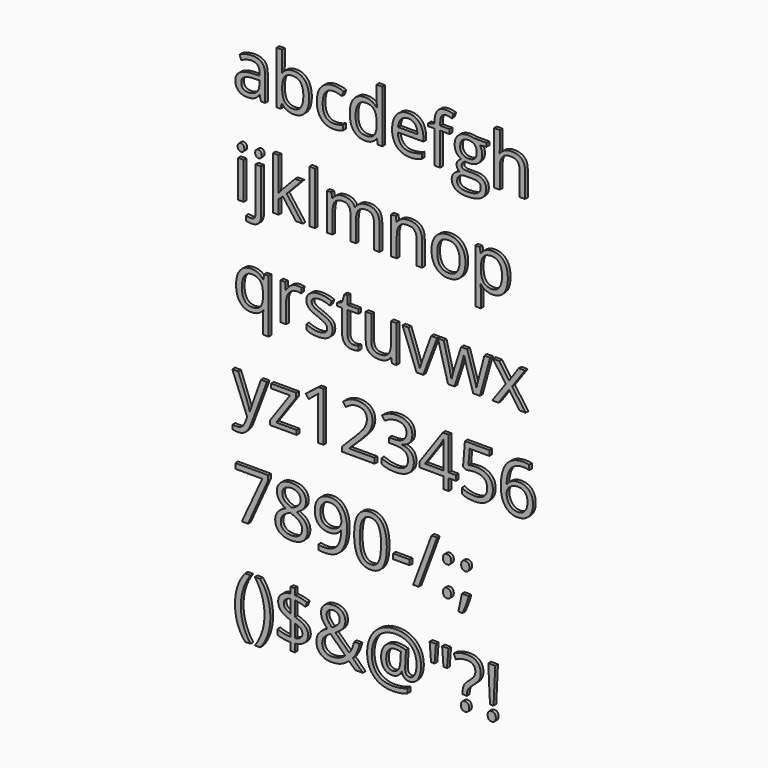
from build123d import *

# Parameters (mm, degrees)
F0_TEXT_SIZE = 508.7015322513
F1_DEPTH     = 25


# Not quite as in the source:
# - Text() gives the source's letters only with a copy of the font that has no kerning and outlines rounded to 1/6400 em; it was checked with that copy


with BuildPart() as f1:
    # F0 (on Front) → F1 (new body)
    with BuildSketch(Plane.XZ):
        with Locations((-146.0869461298, -173.8211065531)):
            Text('abcdefgh', F0_TEXT_SIZE, font='Open Sans', text_align=(TextAlign.LEFT, TextAlign.BOTTOM))
        with Locations((-146.0869461298, -865.6551904149)):
            Text('ijklmnop', F0_TEXT_SIZE, font='Open Sans', text_align=(TextAlign.LEFT, TextAlign.BOTTOM))
        with Locations((-146.0869461298, -1557.4892742766)):
            Text('qrstuvwx', F0_TEXT_SIZE, font='Open Sans', text_align=(TextAlign.LEFT, TextAlign.BOTTOM))
        with Locations((-146.0869461298, -2249.3233581384)):
            Text('yz123456', F0_TEXT_SIZE, font='Open Sans', text_align=(TextAlign.LEFT, TextAlign.BOTTOM))
        with Locations((-146.0869461298, -2941.1574420002)):
            Text('7890-/:;', F0_TEXT_SIZE, font='Open Sans', text_align=(TextAlign.LEFT, TextAlign.BOTTOM))
        with Locations((-146.0869461298, -3632.991525862)):
            Text('()$&@"?!', F0_TEXT_SIZE, font='Open Sans', text_align=(TextAlign.LEFT, TextAlign.BOTTOM))
    extrude(amount=F1_DEPTH)


solid = f1.part
